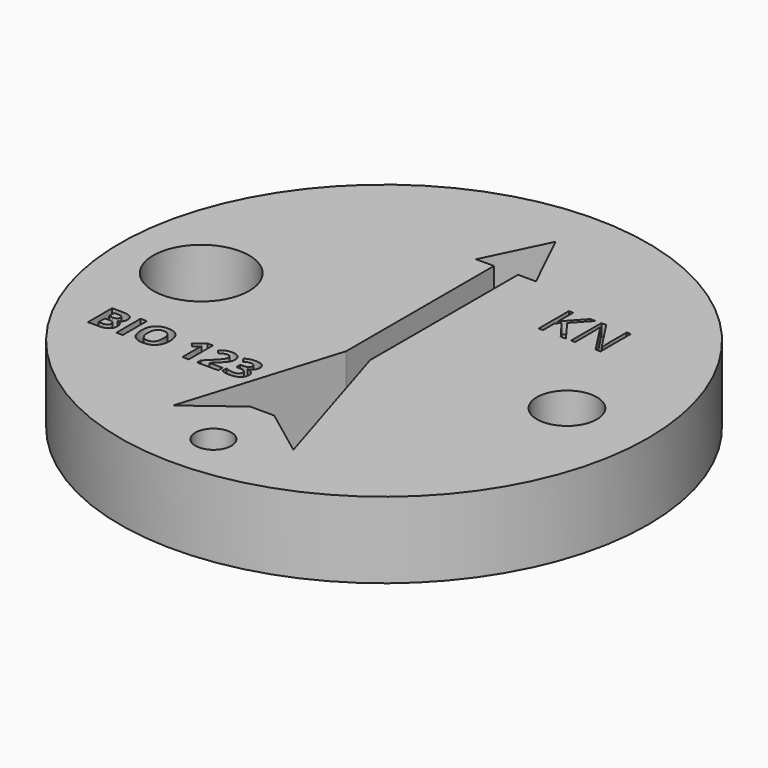
from build123d import *

# Parameters (mm, degrees)
F0_R           = 22
F0_R_2         = 1.5
F0_R_3         = 4
F0_R_4         = 2.5
F1_DEPTH       = 6.35
F2_TEXT_SIZE   = 3.5277777778
F2_TEXT_SIZE_2 = 4.4097222222
F3_DEPTH       = 1


# Not quite as in the source:
# - Text() gives the source's letters only with a copy of the font that has no kerning and outlines rounded to 1/6400 em; it was checked with that copy


with BuildPart() as f1:
    # F0 (on Top) → F1 (new body)
    with BuildSketch(Plane.XY):
        Circle(F0_R)
        with Locations((0, -17.78)):
            Circle(F0_R_2, mode=Mode.SUBTRACT)
        with Locations((-15.24, 0)):
            Circle(F0_R_3, mode=Mode.SUBTRACT)
        Polygon((2.5, 12.7), (1, 12.7), (1, -2.7), (5, -15.7), (1, -12.7), (-1, -12.7), (-5.011445868, -15.6964726771), (-1, -2.7), (-1, 12.7), (-2.5, 12.7), (0, 17.8646296263), align=None, mode=Mode.SUBTRACT)
        with Locations((15.24, 0)):
            Circle(F0_R_4, mode=Mode.SUBTRACT)
    extrude(amount=F1_DEPTH)

    # F2 (on face) → F3 (cut)
    with BuildSketch(Plane.XY.offset(6.35)):
        with Locations((-17, -10)):
            Text('BIO 123', F2_TEXT_SIZE, font='Open Sans', font_style=FontStyle.BOLD, text_align=(TextAlign.LEFT, TextAlign.BOTTOM))
        with Locations((6.35, 7.62)):
            Text('KN', F2_TEXT_SIZE_2, font='Open Sans', text_align=(TextAlign.LEFT, TextAlign.BOTTOM))
    extrude(amount=-F3_DEPTH, mode=Mode.SUBTRACT)


solid = f1.part
